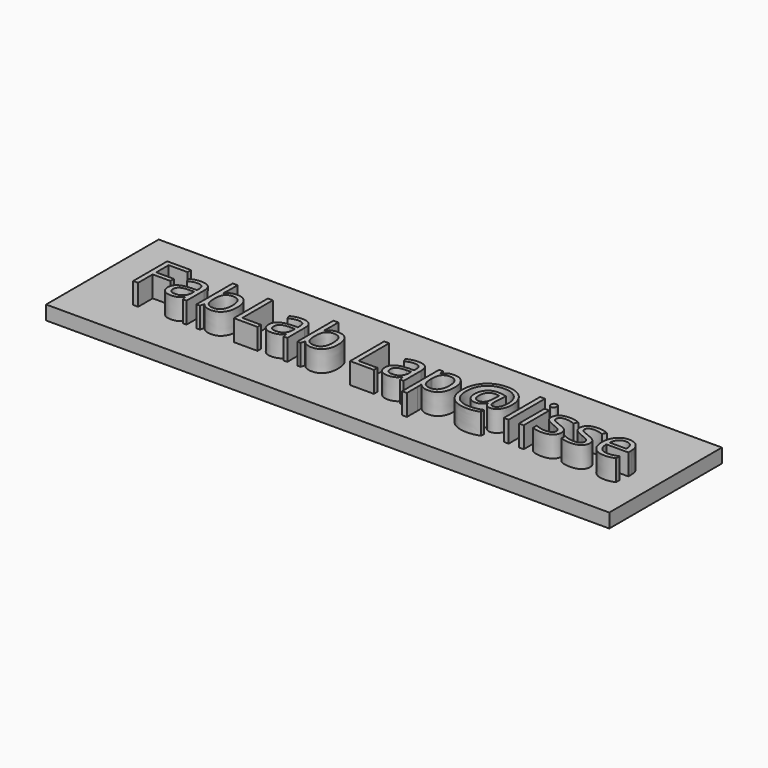
from build123d import *

# Parameters (mm, degrees)
F0_TEXT_SIZE = 8.4814751709
F1_DEPTH     = 3
F2_W         = 80
F2_H         = 20
F3_DEPTH     = 2


# Not quite as in the source:
# - Text() gives the source's letters only with a copy of the font that has no kerning and outlines rounded to 1/6400 em; it was checked with that copy


with BuildPart() as f1:
    # F0 (on Top) → F1 (new body)
    with BuildSketch(Plane.XY):
        with Locations((-1.919152948, -2.4082478752)):
            Text('FabLab Lap@lisse', F0_TEXT_SIZE, font='Open Sans', text_align=(TextAlign.LEFT, TextAlign.BOTTOM))
    extrude(amount=F1_DEPTH)


with BuildPart() as f3:
    # F2 (on Top) → F3 (new body)
    with BuildSketch(Plane.XY):
        with Locations((31.2983173763, 1.6467302585)):
            Rectangle(F2_W, F2_H)
    extrude(amount=-F3_DEPTH)


solid = Compound([f1.part, f3.part])
